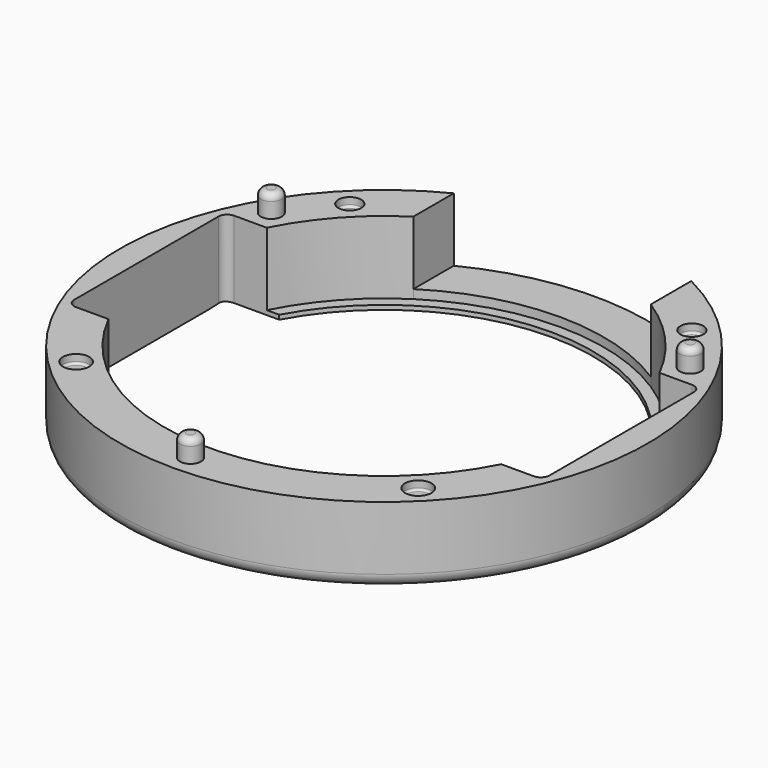
from build123d import *

# Parameters (mm, degrees)
F1_DEPTH  = 17.5
F2_R      = 2.6
F2_R_2    = 3
F3_DEPTH  = 2
F2_R_3    = 2.4
F4_DEPTH  = 5
F5_R      = 0.5
F6_R      = 1.5
F10_DEPTH = 1
F11_DEPTH = 3
F12_R     = 2


# Not quite as in the source:
# - a fillet or chamfer that OpenCascade refuses, or shapes differently, is made with other operations: its cross-section is extruded or revolved along the edge and cut away or added


with BuildPart() as f1:
    # F0 (on Top) → F1 (new body)
    with BuildSketch(Plane.XY):
        with BuildLine():
            ThreePointArc((-27, 53.5817132985), (-31.4642654451, -51.0881590978), (60, 0))
            ThreePointArc((60, 0), (51.0881590978, 31.4642654451), (27, 53.5817132985))
            Line((27, 53.5817132985), (27, 42.083250825))
            ThreePointArc((27, 42.083250825), (37.1397052065, 33.4759958354), (44.6514277487, 22.5))
            Line((44.6514277487, 22.5), (54.0514277487, 22.5))
            Line((54.0514277487, 22.5), (54.0514277487, -22.5))
            Line((54.0514277487, -22.5), (44.6514277487, -22.5))
            ThreePointArc((44.6514277487, -22.5), (0, -50), (-44.6514277487, -22.5))
            Line((-44.6514277487, -22.5), (-54.0514277487, -22.5))
            Line((-54.0514277487, -22.5), (-54.0514277487, 22.5))
            Line((-54.0514277487, 22.5), (-44.6514277487, 22.5))
            ThreePointArc((-44.6514277487, 22.5), (-37.1397052065, 33.4759958354), (-27, 42.083250825))
            Line((-27, 42.083250825), (-27, 53.5817132985))
        make_face()
    extrude(amount=F1_DEPTH)

    # F2 (on face) → F3 (cut)
    with BuildSketch(Plane.XY.offset(17.5)):
        with Locations((-38.8908729653, 38.8908729653)):
            Circle(F2_R)
        with Locations((38.8908729653, 38.8908729653)):
            Circle(F2_R)
        with Locations((38.8908729653, -38.8908729653)):
            Circle(F2_R_2)
        with Locations((-38.8908729653, -38.8908729653)):
            Circle(F2_R_2)
    extrude(amount=-F3_DEPTH, mode=Mode.SUBTRACT)

    # F2 (on face) → F4 (join)
    with BuildSketch(Plane.XY.offset(17.5)):
        with Locations((0, -55)):
            Circle(F2_R_3)
        with Locations((47.6313972081, 27.5)):
            Circle(F2_R_3)
        with Locations((-47.6313972081, 27.5)):
            Circle(F2_R_3)
    extrude(amount=F4_DEPTH)

    # F5
    f5_edges = [f1.edges().sort_by_distance(p)[0] for p in [
        (35.890873, -38.890873, 15.5),
        (-41.890873, -38.890873, 15.5),
        (-41.490873, 38.890873, 15.5),
        (36.290873, 38.890873, 15.5),
    ]]
    fillet(f5_edges, radius=F5_R)

    # F6
    f6_edges = [f1.edges().sort_by_distance(p)[0] for p in [
        (-2.4, -55, 22.5),
        (-50.031397, 27.5, 22.5),
        (45.231397, 27.5, 22.5),
    ]]
    fillet(f6_edges, radius=F6_R)


with BuildPart() as f7_1:
    # F7: copy of F1
    add(f1.part)


with BuildPart() as f1_1:
    add(f1.part)

    # F0 (on Top) → F10 (join)
    with BuildSketch(Plane.XY):
        with BuildLine():
            ThreePointArc((-44.6514277487, -22.5), (0, -50), (44.6514277487, -22.5))
            Line((44.6514277487, -22.5), (41.8330013267, -22.5))
            ThreePointArc((41.8330013267, -22.5), (0, -47.5), (-41.8330013267, -22.5))
            Line((-41.8330013267, -22.5), (-44.6514277487, -22.5))
        make_face()
        with BuildLine():
            ThreePointArc((44.6514277487, 22.5), (37.1397052065, 33.4759958354), (27, 42.083250825))
            ThreePointArc((27, 42.083250825), (0, 50), (-27, 42.083250825))
            ThreePointArc((-27, 42.083250825), (-37.1397052065, 33.4759958354), (-44.6514277487, 22.5))
            Line((-44.6514277487, 22.5), (-41.8330013267, 22.5))
            ThreePointArc((-41.8330013267, 22.5), (0, 47.5), (41.8330013267, 22.5))
            Line((41.8330013267, 22.5), (44.6514277487, 22.5))
        make_face()
    extrude(amount=F10_DEPTH)

    # F0 (on Top) → F11 (join)
    with BuildSketch(Plane.XY):
        with BuildLine():
            Line((27, 42.083250825), (27, 53.5817132985))
            ThreePointArc((27, 53.5817132985), (0, 60), (-27, 53.5817132985))
            Line((-27, 53.5817132985), (-27, 42.083250825))
            ThreePointArc((-27, 42.083250825), (0, 50), (27, 42.083250825))
        make_face()
    extrude(amount=F11_DEPTH)

    # F12
    f12_edges = [f1_1.edges().sort_by_distance(p)[0] for p in [
        (-54.051428, 22.5, 8.75),
        (54.051428, 22.5, 8.75),
        (54.051428, -22.5, 8.75),
        (-54.051428, -22.5, 8.75),
    ]]
    fillet(f12_edges, radius=F12_R)

    # F13: fillet of radius 3 on 1 edges, made by hand

    # F13_s1 → F13_t2 (revolve, cut)
    with BuildSketch(Plane.XZ):
        with BuildLine():
            ThreePointArc((60, 3), (59.1213203436, 0.8786796564), (57, 0))
            Line((57, 0), (60, 0))
            Line((60, 0), (60, 3))
        make_face()
    revolve(axis=Axis((0, 0, 0), (0, 0, 1)), mode=Mode.SUBTRACT)


solid = f1_1.part
